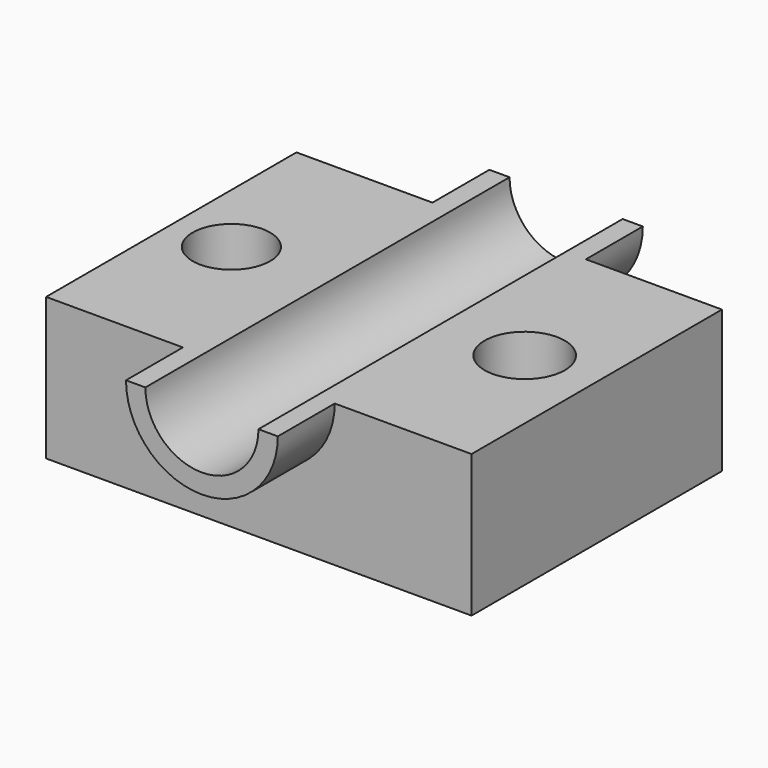
from build123d import *

# Parameters (mm, degrees)
F0_W     = 151.9381850958
F0_H     = 111.7599979043
F0_R     = 13.8333647365
F0_R_2   = 14.3205526474
F1_DEPTH = 50.8
F3_DEPTH = 25.4
F4_DEPTH = 127
F6_DEPTH = 25.4


with BuildPart() as f1:
    # F0 (on Top) → F1 (new body)
    with BuildSketch(Plane.XY):
        with Locations((-0.2309083939, 0.1154541969)):
            Rectangle(F0_W, F0_H)
        with Locations((-54.7254569829, 0.1154541969)):
            Circle(F0_R, mode=Mode.SUBTRACT)
        with Locations((50.1072742045, 0)):
            Circle(F0_R_2, mode=Mode.SUBTRACT)
    extrude(amount=F1_DEPTH)

    # F2 (on face) → F3 (join)
    with BuildSketch(Plane.XZ.offset(55.7645447552)):
        with BuildLine():
            ThreePointArc((-27.3391341012, 50.8), (-0.2309083939, 23.6917742927), (26.8773173135, 50.8))
            Line((26.8773173135, 50.8), (19.9617576881, 50.8))
            ThreePointArc((19.9617576881, 50.8), (-0.2309083939, 30.6073339181), (-20.4235744758, 50.8))
            Line((-20.4235744758, 50.8), (-27.3391341012, 50.8))
        make_face()
    extrude(amount=F3_DEPTH)

    # F4 (cut): a face of the model
    f4_faces = [f1.faces().sort_by_distance(p)[0] for p in [
        (-0.2309083939, -55.7645447552, 42.2299663436),
    ]]
    extrude(f4_faces, amount=-F4_DEPTH, mode=Mode.SUBTRACT)

    # F5 (on face) → F6 (join)
    with BuildSketch(Plane(origin=(0, 55.9954531491, 0), x_dir=(-1, 0, 0), z_dir=(0, 1, 0))):
        with BuildLine():
            ThreePointArc((-27.1668712907, 50.8), (0.2309083939, 23.4022203155), (27.6286880784, 50.8))
            Line((27.6286880784, 50.8), (20.4235744758, 50.8))
            ThreePointArc((20.4235744758, 50.8), (0.2309083939, 30.6073339181), (-19.9617576881, 50.8))
            Line((-19.9617576881, 50.8), (-27.1668712907, 50.8))
        make_face()
    extrude(amount=F6_DEPTH)


solid = f1.part
